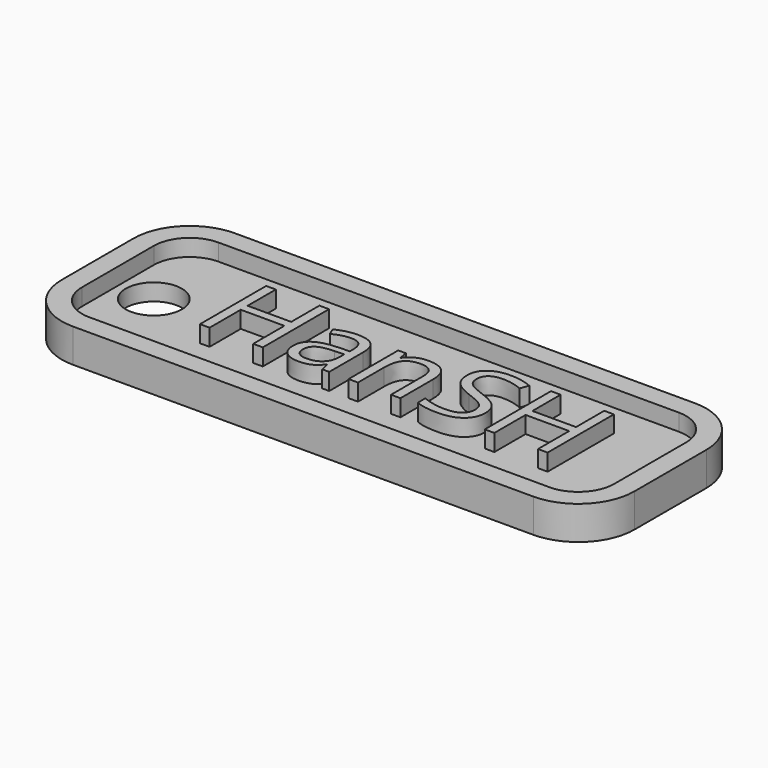
from build123d import *

# Parameters (mm, degrees)
F1_DEPTH     = 1.5
F3_DEPTH     = 1.5
F4_R         = 2.5
F5_DEPTH     = 25
F6_TEXT_SIZE = 10.3250954352
F7_DEPTH     = 1.5


# Not quite as in the source:
# - Text() gives the source's letters only with a copy of the font that has no kerning and outlines rounded to 1/6400 em; it was checked with that copy


with BuildPart() as f1:
    # F0 (on Top) → F1 (new body)
    with BuildSketch(Plane.XY):
        with BuildLine():
            ThreePointArc((0, 5), (1.4644660941, 1.4644660941), (5, 0))
            Line((5, 0), (46, 0))
            ThreePointArc((46, 0), (49.5355339059, 1.4644660941), (51, 5))
            Line((51, 5), (51, 13))
            ThreePointArc((51, 13), (49.5355339059, 16.5355339059), (46, 18))
            Line((46, 18), (5, 18))
            ThreePointArc((5, 18), (1.4644660941, 16.5355339059), (0, 13))
            Line((0, 13), (0, 5))
        make_face()
    extrude(amount=F1_DEPTH)

    # F2 (on face) → F3 (join)
    with BuildSketch(Plane.XY.offset(1.5)):
        with BuildLine():
            Line((0, 13), (0, 5))
            ThreePointArc((0, 5), (1.4644660941, 1.4644660941), (5, 0))
            Line((5, 0), (46, 0))
            ThreePointArc((46, 0), (49.5355339059, 1.4644660941), (51, 5))
            Line((51, 5), (51, 13))
            ThreePointArc((51, 13), (49.5355339059, 16.5355339059), (46, 18))
            Line((46, 18), (5, 18))
            ThreePointArc((5, 18), (1.4644660941, 16.5355339059), (0, 13))
        make_face()
        with BuildLine():
            ThreePointArc((46, 16.2), (48.2627416998, 15.2627416998), (49.2, 13))
            Line((49.2, 13), (49.2, 5))
            ThreePointArc((49.2, 5), (48.2627416998, 2.7372583002), (46, 1.8))
            Line((46, 1.8), (5, 1.8))
            ThreePointArc((5, 1.8), (2.7372583002, 2.7372583002), (1.8, 5))
            Line((1.8, 5), (1.8, 13))
            ThreePointArc((1.8, 13), (2.7372583002, 15.2627416998), (5, 16.2))
            Line((5, 16.2), (46, 16.2))
        make_face(mode=Mode.SUBTRACT)
    extrude(amount=F3_DEPTH)

    # F4 (on face) → F5 (cut)
    with BuildSketch(Plane.XY.offset(1.5)):
        with Locations((5, 9)):
            Circle(F4_R)
    extrude(amount=-F5_DEPTH, mode=Mode.SUBTRACT)

    # F6 (on face) → F7 (join)
    with BuildSketch(Plane.XY.offset(1.5)):
        with Locations((10.6626423076, 5.7935682125)):
            Text('HanSH', F6_TEXT_SIZE, font='Open Sans', text_align=(TextAlign.LEFT, TextAlign.BOTTOM))
    extrude(amount=F7_DEPTH)


solid = f1.part
